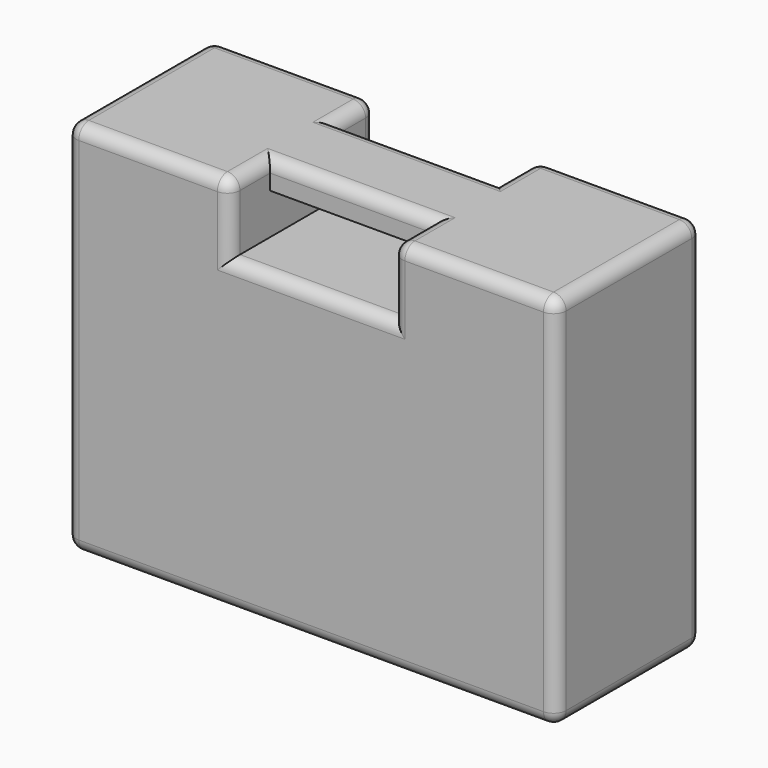
from build123d import *

# Parameters (mm, degrees)
F0_W     = 390
F0_H     = 300
F0_W_2   = 129.2868405581
F0_H_2   = 32.5715690851
F1_DEPTH = 72.5
F2_W     = 129.2868405581
F2_H     = 22.3345696926
F3_DEPTH = 40
F4_R     = 10


# Not quite as in the source:
# - a pattern or mirror of a feature is missing from the dataset's text; its kind, count and spacing are read off the source's solid


with BuildPart() as f1:
    # F0 (on Front) → F1 (new body, symmetric)
    with BuildSketch(Plane.XZ):
        Rectangle(F0_W, F0_H)
        with Locations((0, 111.3796457648)):
            Rectangle(F0_W_2, F0_H_2, mode=Mode.SUBTRACT)
    extrude(amount=F1_DEPTH, both=True)

    # F2 (on face) → F3 (cut)
    with BuildSketch(Plane.XZ.offset(72.5)):
        with Locations((0, 138.8327151537)):
            Rectangle(F2_W, F2_H)
    f3 = extrude(amount=-F3_DEPTH, mode=Mode.SUBTRACT)

    # F3_copies: F3 across plane
    add(f3.mirror(Plane.ZX), mode=Mode.SUBTRACT)

    # F4
    f4_edges = [f1.edges().sort_by_distance(p)[0] for p in [
        (0, -72.5, -150),
        (195, -72.5, 0),
        (129.82171, -72.5, 150),
        (64.64342, -72.5, 122.546931),
        (0, -72.5, 95.093861),
        (-64.64342, -72.5, 122.546931),
        (-129.82171, -72.5, 150),
        (-195, -72.5, 0),
        (-195, 0, 150),
        (-195, 72.5, 0),
        (-195, 0, -150),
        (195, 0, 150),
        (64.64342, -52.5, 150),
        (0, -32.5, 150),
        (-64.64342, -52.5, 150),
        (-129.82171, 72.5, 150),
        (-64.64342, 52.5, 150),
        (0, 32.5, 150),
        (64.64342, 52.5, 150),
        (129.82171, 72.5, 150),
        (0, 72.5, -150),
        (195, 72.5, 0),
        (64.64342, 72.5, 122.546931),
        (0, 72.5, 95.093861),
        (-64.64342, 72.5, 122.546931),
        (195, 0, -150),
    ]]
    fillet(f4_edges, radius=F4_R)


solid = f1.part
